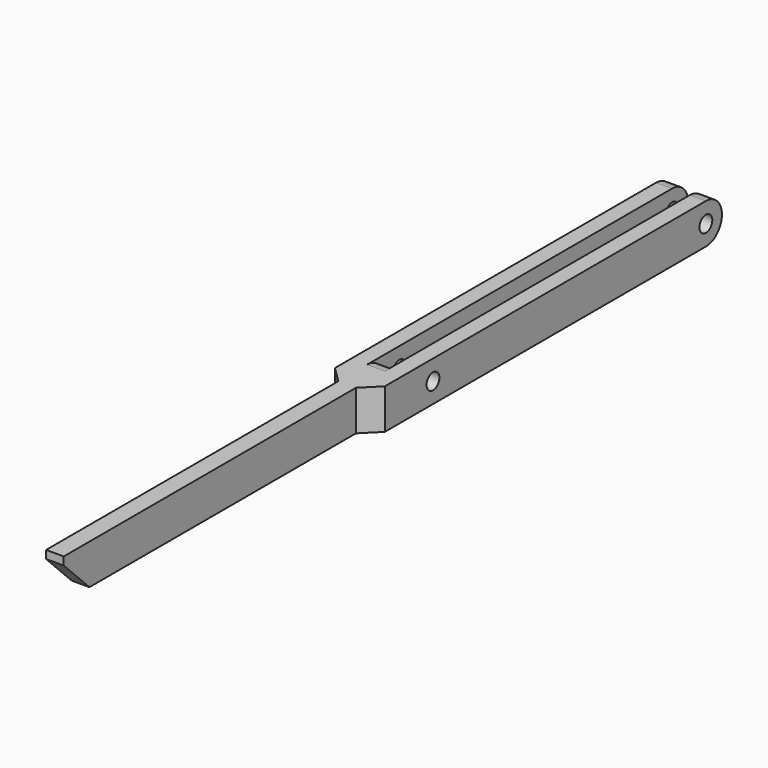
from build123d import *

# Parameters (mm, degrees)
F1_DEPTH      = 2.5
F2_SIZE       = 4
F3_SIZE       = 1.99999
F4_R          = 2.49999
F5_R          = 1
F6_DEPTH      = 3.101
F6_DEPTH_BACK = 3.101


# Not quite as in the source:
# - a fillet or chamfer is up to 0.001 mm smaller than in the source, because OpenCascade refuses the exact size


with BuildPart() as f1:
    # F0 (on Top) → F1 (new body, symmetric)
    with BuildSketch(Plane.XY):
        Polygon((-1.1, -50), (0, -50), (1.1, -50), (1.1, -2.5), (3.1, -2.5), (3.1, 50), (1.1, 50), (1.1, 2.5), (0, 2.5), (-1.1, 2.5), (-1.1, 50), (-3.1, 50), (-3.1, -2.5), (-1.1, -2.5), align=None)
    extrude(amount=F1_DEPTH, both=True)

    # F2
    f2_edges = [f1.edges().sort_by_distance(p)[0] for p in [
        (0, -50, -2.5),
    ]]
    chamfer(f2_edges, length=F2_SIZE)

    # F3 (size 2 in the source; OpenCascade refuses exactly that, so slightly less here)
    f3_edges = [f1.edges().sort_by_distance(p)[0] for p in [
        (1.1, -2.5, 0),
        (-1.1, -2.5, 0),
    ]]
    chamfer(f3_edges, length=F3_SIZE)

    # F4 (radius 2.5 in the source; OpenCascade refuses exactly that, so slightly less here)
    f4_edges = [f1.edges().sort_by_distance(p)[0] for p in [
        (2.1, 50, 2.5),
        (-2.1, 50, 2.5),
        (-2.1, 50, -2.5),
        (2.1, 50, -2.5),
        (0, 2.5, -2.5),
        (0, 2.5, 2.5),
    ]]
    fillet(f4_edges, radius=F4_R)

    # F5 (on Right) → F6 (cut, two sides)
    with BuildSketch(Plane.YZ) as f6_sk:
        with Locations((5, 0)):
            Circle(F5_R)
        with Locations((47.5, 0)):
            Circle(F5_R)
    extrude(amount=-F6_DEPTH, mode=Mode.SUBTRACT)
    extrude(f6_sk.sketch, amount=F6_DEPTH_BACK, mode=Mode.SUBTRACT)


solid = f1.part
